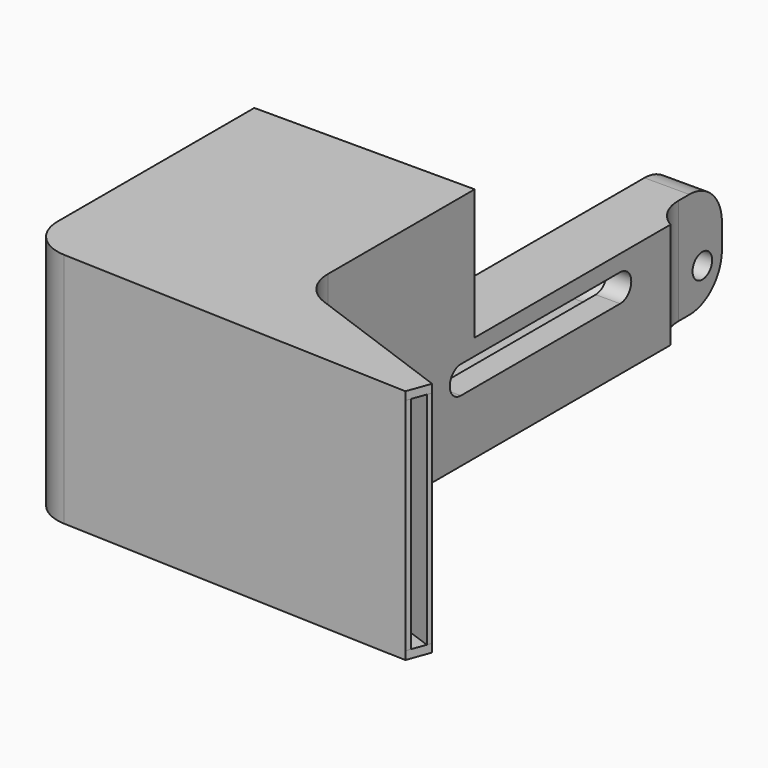
from build123d import *

# Parameters (mm, degrees)
F1_DEPTH      = 1
F3_DEPTH      = 27
F5_DEPTH      = 1
F7_DEPTH      = 13
F8_R          = 1.5
F9_DEPTH      = 25
F10_DEPTH     = 5
F11_T1_DEPTH  = 29
F11_T3_DEPTH  = 13
F11_T5_DEPTH  = 27
F11_T7_DEPTH  = 30.5
F11_T9_DEPTH  = 30.5
F11_T11_DEPTH = 53.0467878714
F11_T13_DEPTH = 27


# Not quite as in the source:
# - a fillet or chamfer that OpenCascade refuses, or shapes differently, is made with other operations: its cross-section is extruded or revolved along the edge and cut away or added


with BuildPart() as f1:
    # F0 (on Top) → F1 (new body)
    with BuildSketch(Plane.XY):
        Polygon((0, 34.9576839236), (0, 0), (47.9637535727, -1.8650316928), (48.9898140027, 0.9540461696), (27, 8.9576839236), (27, 34.9576839236), align=None)
    extrude(amount=F1_DEPTH)

    # F2 (on face) → F3 (join)
    with BuildSketch(Plane.XY.offset(1)):
        Polygon((2.5, 34.9576839236), (0, 34.9576839236), (0, 0), (47.9637535727, -1.8650316928), (48.1792508796, -1.2729577082), (2.5, 0.5032429485), align=None)
        Polygon((27, 34.9576839236), (19, 34.9576839236), (19, 11.2309391343), (48.7846019167, 0.3902305971), (48.9898140027, 0.9540461696), (27, 8.9576839236), align=None)
    extrude(amount=F3_DEPTH)

    # F4 (on face) → F5 (join)
    with BuildSketch(Plane.XY.offset(28)):
        Polygon((0, 34.9576839236), (0, 0), (47.9637535727, -1.8650316928), (48.9898140027, 0.9540461696), (27, 8.9576839236), (27, 34.9576839236), align=None)
    extrude(amount=F5_DEPTH)

    # F6 (on face) → F7 (join)
    with BuildSketch(Plane(origin=(0, 0, 0), x_dir=(1, 0, 0), z_dir=(0, 0, -1))):
        Polygon((27, -64.9576839236), (27, -34.9576839236), (19, -34.9576839236), (19, -75.9576839236), (24.5, -75.9576839236), (24.5, -64.9576839236), align=None)
    extrude(amount=-F7_DEPTH)

    # F8 (on face) → F9 (cut)
    with BuildSketch(Plane(origin=(19, 0, 0), x_dir=(0, -1, 0), z_dir=(-1, 0, 0))):
        with Locations((-72.9576839236, 4.5)):
            Circle(F8_R)
        with BuildLine():
            Line((-32.8452885151, 11), (-57.2458393872, 11))
            ThreePointArc((-57.2458393872, 11), (-58.9458393872, 9.3), (-57.2458393872, 7.6))
            Line((-57.2458393872, 7.6), (-32.8452885151, 7.6))
            ThreePointArc((-32.8452885151, 7.6), (-31.1452885151, 9.3), (-32.8452885151, 11))
        make_face()
    extrude(amount=-F9_DEPTH, mode=Mode.SUBTRACT)

    # F8 (on face) → F10 (cut)
    with BuildSketch(Plane(origin=(19, 0, 0), x_dir=(0, -1, 0), z_dir=(-1, 0, 0))):
        with BuildLine():
            Line((-32.8452885151, 12.3), (-57.2458393872, 12.3))
            ThreePointArc((-57.2458393872, 12.3), (-60.2458393872, 9.3), (-57.2458393872, 6.3))
            Line((-57.2458393872, 6.3), (-32.8452885151, 6.3))
            ThreePointArc((-32.8452885151, 6.3), (-29.8452885151, 9.3), (-32.8452885151, 12.3))
        make_face()
        with BuildLine():
            ThreePointArc((-57.2458393872, 7.6), (-58.9458393872, 9.3), (-57.2458393872, 11))
            Line((-57.2458393872, 11), (-32.8452885151, 11))
            ThreePointArc((-32.8452885151, 11), (-31.1452885151, 9.3), (-32.8452885151, 7.6))
            Line((-32.8452885151, 7.6), (-57.2458393872, 7.6))
        make_face(mode=Mode.SUBTRACT)
    extrude(amount=-F10_DEPTH, mode=Mode.SUBTRACT)

    # F11: fillet of radius 5 on 7 edges, made by hand

    # F11_s2 → F11_t1 (join)
    with BuildSketch(Plane.XY):
        with BuildLine():
            ThreePointArc((27, 12.4587216147), (27.9042397786, 9.5908394329), (30.2898992834, 7.7602585108))
            Line((30.2898992834, 7.7602585108), (27, 8.9576839236))
            Line((27, 8.9576839236), (27, 12.4587216147))
        make_face()
    extrude(amount=F11_T1_DEPTH)

    # F11_s4 → F11_t3 (join)
    with BuildSketch(Plane.XY):
        with BuildLine():
            ThreePointArc((27, 64.9576839236), (25.1698729811, 66.7878109426), (24.5, 69.2878109426))
            Line((24.5, 69.2878109426), (24.5, 64.9576839236))
            Line((24.5, 64.9576839236), (27, 64.9576839236))
        make_face()
    extrude(amount=F11_T3_DEPTH)

    # F11_s6 → F11_t5 (join)
    with BuildSketch(Plane.XY.offset(1)):
        with BuildLine():
            ThreePointArc((2.5, 5.3126005228), (3.8964343579, 1.8464333797), (7.3057258653, 0.3163761923))
            Line((7.3057258653, 0.3163761923), (2.5, 0.5032429485))
            Line((2.5, 0.5032429485), (2.5, 5.3126005228))
        make_face()
    extrude(amount=F11_T5_DEPTH)

    # F11_s8 → F11_t7 (cut)
    with BuildSketch(Plane.YZ.offset(6.5)):
        with BuildLine():
            ThreePointArc((70.9576839236, 0), (74.4932178296, 1.4644660941), (75.9576839236, 5))
            Line((75.9576839236, 5), (75.9576839236, 0))
            Line((75.9576839236, 0), (70.9576839236, 0))
        make_face()
    extrude(amount=F11_T7_DEPTH, mode=Mode.SUBTRACT)

    # F11_s10 → F11_t9 (cut)
    with BuildSketch(Plane.YZ.offset(6.5)):
        with BuildLine():
            ThreePointArc((70.9576839236, 13), (74.4932178296, 11.5355339059), (75.9576839236, 8))
            Line((75.9576839236, 8), (75.9576839236, 13))
            Line((75.9576839236, 13), (70.9576839236, 13))
        make_face()
    extrude(amount=F11_T9_DEPTH, mode=Mode.SUBTRACT)

    # F11_s12 → F11_t11 (cut)
    with BuildSketch(Plane.XY.offset(-12.0233939357)):
        with BuildLine():
            ThreePointArc((4.8057258653, -0.1868667562), (1.3964343579, 1.3431904313), (0, 4.8093575743))
            Line((0, 4.8093575743), (0, 0))
            Line((0, 0), (4.8057258653, -0.1868667562))
        make_face()
    extrude(amount=F11_T11_DEPTH, mode=Mode.SUBTRACT)

    # F11_s14 → F11_t13 (cut)
    with BuildSketch(Plane.XY.offset(1)):
        with BuildLine():
            ThreePointArc((19, 14.7319768253), (19.9042397786, 11.8640946436), (22.2898992834, 10.0335137214))
            Line((22.2898992834, 10.0335137214), (19, 11.2309391343))
            Line((19, 11.2309391343), (19, 14.7319768253))
        make_face()
    extrude(amount=F11_T13_DEPTH, mode=Mode.SUBTRACT)


solid = f1.part
